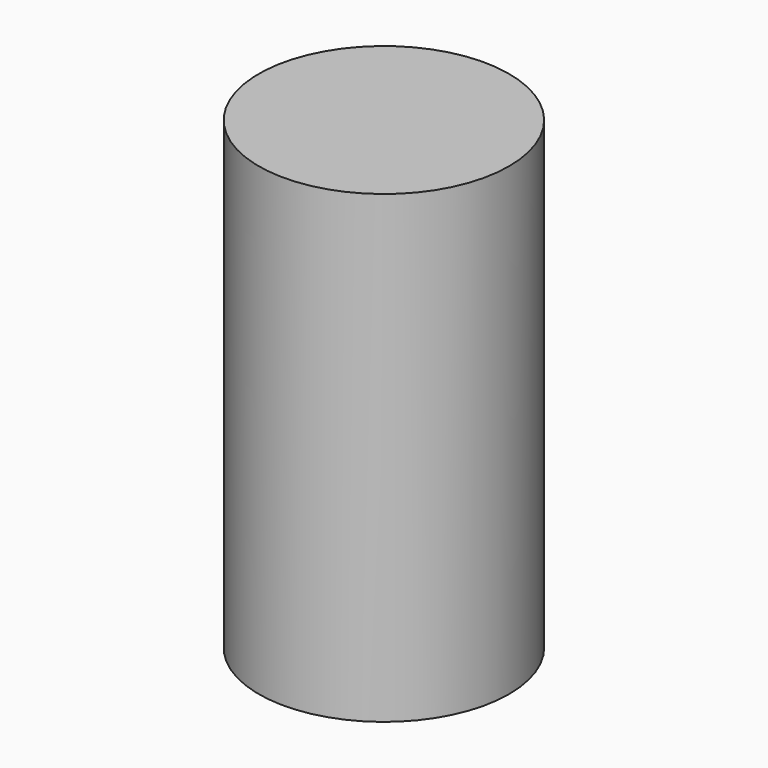
from build123d import *

# Parameters (mm, degrees)
F0_R     = 18.85
F0_R_2   = 15.85
F1_DEPTH = 70
F4_R     = 18.85
F5_REACH = 97.9158513015


with BuildPart() as f1:
    # F0 (on Top) → F1 (new body)
    with BuildSketch(Plane.XY):
        Circle(F0_R)
        Circle(F0_R_2, mode=Mode.SUBTRACT)
    extrude(amount=-F1_DEPTH)

    f5_end = Plane(origin=(-14.1617017286, 0, -16.8421500054), x_dir=(0.7653848138, 0, -0.6435729071), z_dir=(0.6435729071, 0, 0.7653848138))
    # F4 (on face) → F5 (join, up to a plane its end follows)
    with BuildSketch(Plane.XY):
        Circle(F4_R)
    f5_long = extrude(amount=-F5_REACH, mode=Mode.PRIVATE)
    add(split(f5_long, bisect_by=f5_end, keep=Keep.TOP, mode=Mode.PRIVATE))


solid = f1.part
